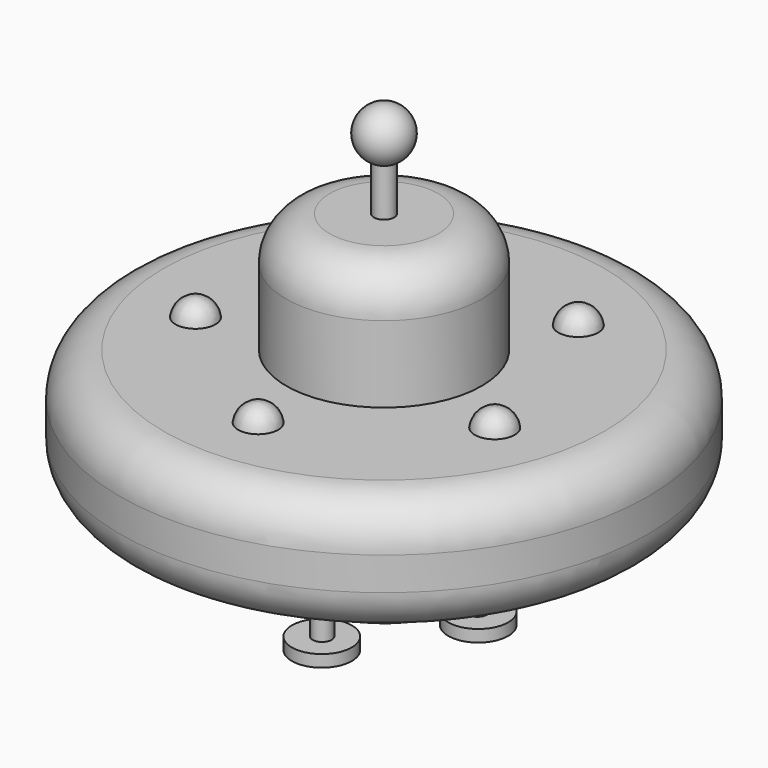
from build123d import *

# Parameters (mm, degrees)
F0_R      = 55.907699691
F0_R_2    = 20.7094261491
F1_DEPTH  = 25.4
F2_DEPTH  = 50.8
F3_R      = 9.1981536726
F4_R      = 11.7499881289
F5_DEPTH  = 14.986
F7_R      = 2.155396083
F8_DEPTH  = 11.176
F13_R     = 2.0110469696
F14_DEPTH = 6.858
F15_R     = 6.35
F15_R_2   = 2.0110469696
F16_DEPTH = 2.54
F17_R     = 4.2250159327
F18_DEPTH = 3.81


# Not quite as in the source:
# - a fillet or chamfer that OpenCascade refuses, or shapes differently, is made with other operations: its cross-section is extruded or revolved along the edge and cut away or added


with BuildPart() as f1:
    # F0 (on Top) → F1 (new body)
    with BuildSketch(Plane.XY):
        Circle(F0_R)
        Circle(F0_R_2, mode=Mode.SUBTRACT)
    extrude(amount=F1_DEPTH)

    # F0 (on Top) → F2 (join)
    with BuildSketch(Plane.XY):
        Circle(F0_R_2)
    extrude(amount=F2_DEPTH)

    # F3
    f3_edges = [f1.edges().sort_by_distance(p)[0] for p in [
        (-55.9077, 0, 25.4),
        (-55.9077, 0, 0),
        (-20.709426, 0, 50.8),
    ]]
    fillet(f3_edges, radius=F3_R)

    # F4 (on Top) → F5 (join)
    with BuildSketch(Plane.XY):
        with BuildLine():
            ThreePointArc((0, -20.4209801223), (14.4398135229, -14.4398135229), (20.4209801223, 0))
            ThreePointArc((20.4209801223, 0), (-14.4398135229, 14.4398135229), (0, -20.4209801223))
        make_face()
        Circle(F4_R, mode=Mode.SUBTRACT)
    extrude(amount=-F5_DEPTH)

    # F7 (on offset) → F8 (join)
    with BuildSketch(Plane.XY.offset(50.8)):
        Circle(F7_R)
    extrude(amount=F8_DEPTH)


with BuildPart() as f10:
    # F9 (on Front) → F10 (revolve)
    with BuildSketch(Plane.XZ):
        with BuildLine():
            Line((0, 60.3753858651), (0, 71.263006941))
            ThreePointArc((0, 71.263006941), (-5.4438105379, 65.819196403), (0, 60.3753858651))
        make_face()
    revolve(axis=Axis((0, 0, 65.819196403), (0, 0, -1)))


with BuildPart() as f12:
    # F11 (on Front) → F12 (revolve)
    with BuildSketch(Plane.XZ):
        Polygon((20.4697810113, 0), (20.4697810113, -13.023798354), (44.8134429753, 0), align=None)
    revolve(axis=Axis((0, 0, 0), (0, 0, 1)))


with BuildPart() as f14:
    # F13 (on face) → F14 (new body)
    with BuildSketch(Plane(origin=(0, 0, -14.986), x_dir=(1, 0, 0), z_dir=(0, 0, -1))):
        with Locations((-13.3143390791, -8.3219271139)):
            Circle(F13_R)
    extrude(amount=F14_DEPTH)


with BuildPart() as f14b:
    # F13 (on face) → F14, piece 2 (new body)
    with BuildSketch(Plane(origin=(0, 0, -14.986), x_dir=(1, 0, 0), z_dir=(0, 0, -1))):
        with Locations((-0.5498307495, 15.691519434)):
            Circle(F13_R)
    extrude(amount=F14_DEPTH)


with BuildPart() as f14c:
    # F13 (on face) → F14, piece 3 (new body)
    with BuildSketch(Plane(origin=(0, 0, -14.986), x_dir=(1, 0, 0), z_dir=(0, 0, -1))):
        with Locations((13.8641698286, -7.3695923202)):
            Circle(F13_R)
    extrude(amount=F14_DEPTH)


with BuildPart() as f16:
    # F15 (on face) → F16 (new body)
    with BuildSketch(Plane(origin=(0, 0, -21.844), x_dir=(1, 0, 0), z_dir=(0, 0, -1))):
        with Locations((-13.3143390791, -8.3219271139)):
            Circle(F15_R)
        with Locations((-13.3143390791, -8.3219271139)):
            Circle(F15_R_2, mode=Mode.SUBTRACT)
        with Locations((-13.3143390791, -8.3219271139)):
            Circle(F15_R_2)
    extrude(amount=F16_DEPTH)


with BuildPart() as f16b:
    # F15 (on face) → F16, piece 2 (new body)
    with BuildSketch(Plane(origin=(0, 0, -21.844), x_dir=(1, 0, 0), z_dir=(0, 0, -1))):
        with Locations((14.0013098717, -7.4643460102)):
            Circle(F15_R)
    extrude(amount=F16_DEPTH)


with BuildPart() as f16c:
    # F15 (on face) → F16, piece 3 (new body)
    with BuildSketch(Plane(origin=(0, 0, -21.844), x_dir=(1, 0, 0), z_dir=(0, 0, -1))):
        with Locations((-0.5914923968, 15.7245695591)):
            Circle(F15_R)
    extrude(amount=F16_DEPTH)


with BuildPart() as f18:
    # F17 (on face) → F18 (new body)
    with BuildSketch(Plane.XY.offset(25.4)):
        with Locations((0, -33.3297215402)):
            Circle(F17_R)
    extrude(amount=F18_DEPTH)

    # F19: fillet of radius 4.22402 on 1 edges, made by hand

    # F19_s1 → F19_t2 (revolve, cut)
    with BuildSketch(Plane.XZ.offset(33.3297215402)):
        with BuildLine():
            ThreePointArc((4.2250159327, 25.4), (2.8580159415, 28.1157702263), (0.021335117, 29.21))
            Line((0.021335117, 29.21), (4.2250159327, 29.21))
            Line((4.2250159327, 29.21), (4.2250159327, 25.4))
        make_face()
    revolve(axis=Axis((0, -33.3297215402, 29.21), (0, 0, 1)), mode=Mode.SUBTRACT)


with BuildPart() as f18b:
    # F17 (on face) → F18, piece 2 (new body)
    with BuildSketch(Plane.XY.offset(25.4)):
        with Locations((31.6984488571, -10.2994503737)):
            Circle(F17_R)
    extrude(amount=F18_DEPTH)

    # F19#2: fillet of radius 4.22402 on 1 edges, made by hand

    # F19_2_s1 → F19_2_t2 (revolve, cut)
    with BuildSketch(Plane.XZ.offset(10.2994503737)):
        with BuildLine():
            ThreePointArc((35.9234647898, 25.4), (34.5564647986, 28.1157702263), (31.7197839742, 29.21))
            Line((31.7197839742, 29.21), (35.9234647898, 29.21))
            Line((35.9234647898, 29.21), (35.9234647898, 25.4))
        make_face()
    revolve(axis=Axis((31.6984488571, -10.2994503737, 29.21), (0, 0, 1)), mode=Mode.SUBTRACT)


with BuildPart() as f18c:
    # F17 (on face) → F18, piece 3 (new body)
    with BuildSketch(Plane.XY.offset(25.4)):
        with Locations((19.5907187844, 26.9643111438)):
            Circle(F17_R)
    extrude(amount=F18_DEPTH)

    # F19#3: fillet of radius 4.22402 on 1 edges, made by hand

    # F19_3_s1 → F19_3_t2 (revolve, cut)
    with BuildSketch(Plane.XZ.offset(-26.9643111438)):
        with BuildLine():
            ThreePointArc((23.815734717, 25.4), (22.4487347259, 28.1157702263), (19.6120539014, 29.21))
            Line((19.6120539014, 29.21), (23.815734717, 29.21))
            Line((23.815734717, 29.21), (23.815734717, 25.4))
        make_face()
    revolve(axis=Axis((19.5907187844, 26.9643111438, 29.21), (0, 0, 1)), mode=Mode.SUBTRACT)


with BuildPart() as f18d:
    # F17 (on face) → F18, piece 4 (new body)
    with BuildSketch(Plane.XY.offset(25.4)):
        with Locations((-19.5907187844, 26.9643111438)):
            Circle(F17_R)
    extrude(amount=F18_DEPTH)

    # F19#4: fillet of radius 4.22402 on 1 edges, made by hand

    # F19_4_s1 → F19_4_t2 (revolve, cut)
    with BuildSketch(Plane.XZ.offset(-26.9643111438)):
        with BuildLine():
            ThreePointArc((-15.3657028517, 25.4), (-16.7327028428, 28.1157702263), (-19.5693836673, 29.21))
            Line((-19.5693836673, 29.21), (-15.3657028517, 29.21))
            Line((-15.3657028517, 29.21), (-15.3657028517, 25.4))
        make_face()
    revolve(axis=Axis((-19.5907187844, 26.9643111438, 29.21), (0, 0, 1)), mode=Mode.SUBTRACT)


with BuildPart() as f18e:
    # F17 (on face) → F18, piece 5 (new body)
    with BuildSketch(Plane.XY.offset(25.4)):
        with Locations((-31.6984488571, -10.2994503737)):
            Circle(F17_R)
    extrude(amount=F18_DEPTH)

    # F19#5: fillet of radius 4.22402 on 1 edges, made by hand

    # F19_5_s1 → F19_5_t2 (revolve, cut)
    with BuildSketch(Plane.XZ.offset(10.2994503737)):
        with BuildLine():
            ThreePointArc((-27.4734329244, 25.4), (-28.8404329156, 28.1157702263), (-31.6771137401, 29.21))
            Line((-31.6771137401, 29.21), (-27.4734329244, 29.21))
            Line((-27.4734329244, 29.21), (-27.4734329244, 25.4))
        make_face()
    revolve(axis=Axis((-31.6984488571, -10.2994503737, 29.21), (0, 0, 1)), mode=Mode.SUBTRACT)


solid = Compound([f1.part, f10.part, f12.part, f14.part, f14b.part, f14c.part, f16.part, f16b.part, f16c.part, f18.part, f18b.part, f18c.part, f18d.part, f18e.part])
